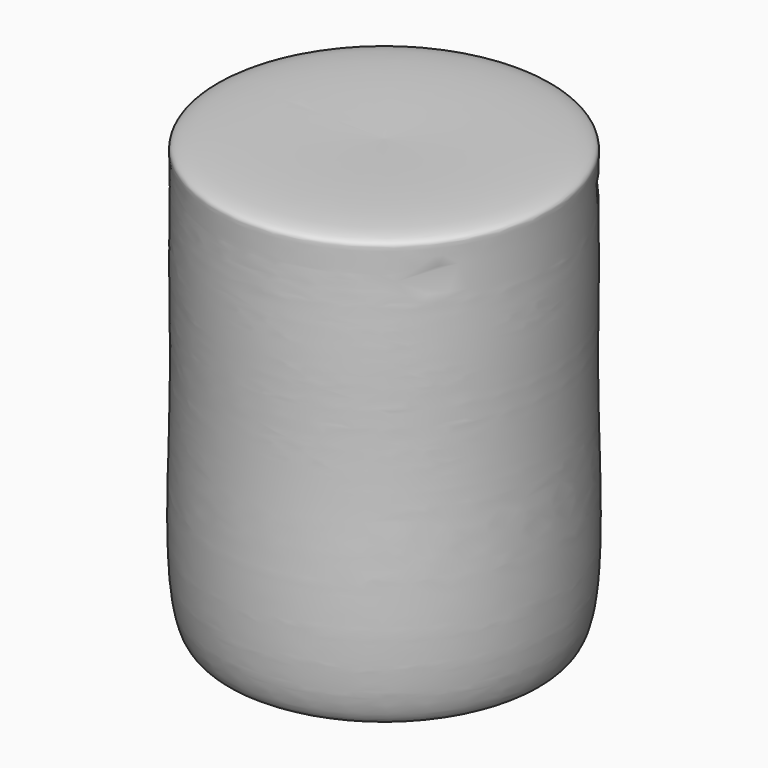
from build123d import *


# Not quite as in the source:
# - the program builds the solid bodies; features that only make, move or delete a surface that nothing else refers to are left out


with BuildPart() as f1:
    # F0 (on Front) → F1 (revolve)
    with BuildSketch(Plane.XZ):
        with BuildLine():
            add(Edge.make_bspline(
                [(0, 0), (-7.0481867769, 0.4614734699), (-17.9880833627, 1.1777530178), (-27.6470794563, -3.5474272712), (-26.0065526211, 31.8387677014), (-26.5457101991, 48.6464645431), (-26.2527485063, 65.1647899221), (-26.7505995854, 68.4900627658), (-11.8692267951, 68.1295736907), (0, 67.8420513868)],
                knots=[0, 0, 0, 0, 0.1606031179, 0.2492813481, 0.4497418218, 0.6216953011, 0.7635804795, 0.8114342711, 1, 1, 1, 1], degree=3))
            Line((0, 0), (0, 67.8420513868))
        make_face()
    revolve(axis=Axis((0, 0, 39.775416255), (0, 0, 1)))


solid = f1.part
